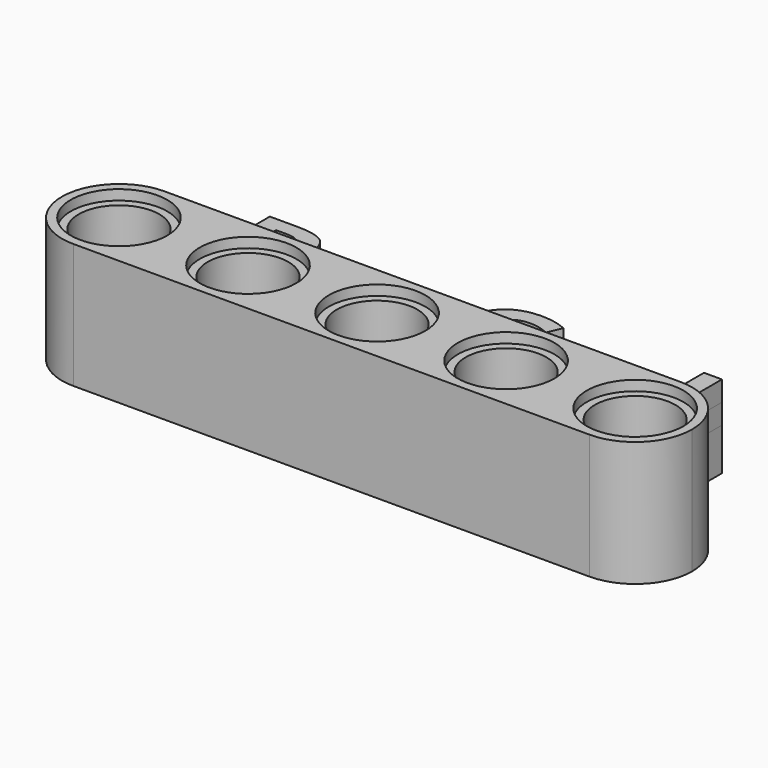
from build123d import *

# Parameters (mm, degrees)
F0_R         = 3.048
F0_R_2       = 2.54
F1_DEPTH     = 3.937
F2_R         = 3.0417071759
F3_DEPTH     = 0.635
F4_R         = 3.048
F5_DEPTH     = 0.635
F6_TEXT_SIZE = 7.5637000716
F7_DEPTH     = 3.937
F8_SIZE2     = 0.50799
F8_SIZE      = 0.50799
F9_SIZE2     = 0.50799
F9_SIZE      = 0.50799
F10_DEPTH    = 1.27


# Not quite as in the source:
# - a fillet or chamfer is up to 0.001 mm smaller than in the source, because OpenCascade refuses the exact size
# - Text() gives the source's letters only with a copy of the font that has no kerning and outlines rounded to 1/6400 em; it was checked with that copy


with BuildPart() as f1:
    # F0 (on Top) → F1 (new body, symmetric)
    with BuildSketch(Plane.XY):
        with BuildLine():
            ThreePointArc((-40.9946195992, 14.3710068385), (-42.0464330806, 16.9103092103), (-44.5857354524, 17.9621226917))
            ThreePointArc((-44.5857354524, 17.9621226917), (-48.1768513056, 14.3710068385), (-44.5857354524, 10.7798909853))
            ThreePointArc((-44.5857354524, 10.7798909853), (-42.0464330806, 11.8317044667), (-40.9946195992, 14.3710068385))
        make_face()
        with Locations((-44.5857354524, 14.3710068385)):
            Circle(F0_R, mode=Mode.SUBTRACT)
        with BuildLine():
            ThreePointArc((-49.1226195992, 14.3710068385), (-50.1744330806, 16.9103092103), (-52.7137354524, 17.9621226917))
            ThreePointArc((-52.7137354524, 17.9621226917), (-56.3048513056, 14.3710068385), (-52.7137354524, 10.7798909853))
            ThreePointArc((-52.7137354524, 10.7798909853), (-50.1744330806, 11.8317044667), (-49.1226195992, 14.3710068385))
        make_face()
        with Locations((-52.7137354524, 14.3710068385)):
            Circle(F0_R, mode=Mode.SUBTRACT)
        with BuildLine():
            ThreePointArc((-32.8666195992, 14.3710068385), (-33.9184330806, 16.9103092103), (-36.4577354524, 17.9621226917))
            ThreePointArc((-36.4577354524, 17.9621226917), (-40.0488513056, 14.3710068385), (-36.4577354524, 10.7798909853))
            ThreePointArc((-36.4577354524, 10.7798909853), (-33.9184330806, 11.8317044667), (-32.8666195992, 14.3710068385))
        make_face()
        with Locations((-36.4577354524, 14.3710068385)):
            Circle(F0_R, mode=Mode.SUBTRACT)
        with BuildLine():
            ThreePointArc((-24.7386195992, 14.3710068385), (-25.7904330806, 16.9103092103), (-28.3297354524, 17.9621226917))
            ThreePointArc((-28.3297354524, 17.9621226917), (-31.9208513056, 14.3710068385), (-28.3297354524, 10.7798909853))
            ThreePointArc((-28.3297354524, 10.7798909853), (-25.7904330806, 11.8317044667), (-24.7386195992, 14.3710068385))
        make_face()
        with Locations((-28.3297354524, 14.3710068385)):
            Circle(F0_R, mode=Mode.SUBTRACT)
        with BuildLine():
            ThreePointArc((-60.8417354524, 10.7798909853), (-58.3024330806, 11.8317044667), (-57.2506195992, 14.3710068385))
            ThreePointArc((-57.2506195992, 14.3710068385), (-58.3024330806, 16.9103092103), (-60.8417354524, 17.9621226917))
            ThreePointArc((-60.8417354524, 17.9621226917), (-64.4328513056, 14.3710068385), (-60.8417354524, 10.7798909853))
        make_face()
        with Locations((-60.8417354524, 14.3710068385)):
            Circle(F0_R, mode=Mode.SUBTRACT)
        with Locations((-44.5857354524, 14.3710068385)):
            Circle(F0_R)
        with Locations((-44.5857354524, 14.3710068385)):
            Circle(F0_R_2, mode=Mode.SUBTRACT)
        with Locations((-36.4577354524, 14.3710068385)):
            Circle(F0_R)
        with Locations((-36.4577354524, 14.3710068385)):
            Circle(F0_R_2, mode=Mode.SUBTRACT)
        with Locations((-52.7137354524, 14.3710068385)):
            Circle(F0_R)
        with Locations((-52.7137354524, 14.3710068385)):
            Circle(F0_R_2, mode=Mode.SUBTRACT)
        with Locations((-28.3297354524, 14.3710068385)):
            Circle(F0_R)
        with Locations((-28.3297354524, 14.3710068385)):
            Circle(F0_R_2, mode=Mode.SUBTRACT)
        with Locations((-60.8417354524, 14.3710068385)):
            Circle(F0_R)
        with Locations((-60.8417354524, 14.3710068385)):
            Circle(F0_R_2, mode=Mode.SUBTRACT)
        with BuildLine():
            ThreePointArc((-60.8417354524, 17.9621226917), (-58.3024330806, 16.9103092103), (-57.2506195992, 14.3710068385))
            ThreePointArc((-57.2506195992, 14.3710068385), (-58.3024330806, 11.8317044667), (-60.8417354524, 10.7798909853))
            Line((-60.8417354524, 10.7798909853), (-52.7137354524, 10.7798909853))
            ThreePointArc((-52.7137354524, 10.7798909853), (-56.3048513056, 14.3710068385), (-52.7137354524, 17.9621226917))
            Line((-52.7137354524, 17.9621226917), (-60.8417354524, 17.9621226917))
        make_face()
        with BuildLine():
            Line((-44.5857354524, 17.9621226917), (-52.7137354524, 17.9621226917))
            ThreePointArc((-52.7137354524, 17.9621226917), (-50.1744330806, 16.9103092103), (-49.1226195992, 14.3710068385))
            ThreePointArc((-49.1226195992, 14.3710068385), (-50.1744330806, 11.8317044667), (-52.7137354524, 10.7798909853))
            Line((-52.7137354524, 10.7798909853), (-44.5857354524, 10.7798909853))
            ThreePointArc((-44.5857354524, 10.7798909853), (-48.1768513056, 14.3710068385), (-44.5857354524, 17.9621226917))
        make_face()
        with BuildLine():
            Line((-28.3297354524, 17.9621226917), (-36.4577354524, 17.9621226917))
            ThreePointArc((-36.4577354524, 17.9621226917), (-33.9184330806, 16.9103092103), (-32.8666195992, 14.3710068385))
            ThreePointArc((-32.8666195992, 14.3710068385), (-33.9184330806, 11.8317044667), (-36.4577354524, 10.7798909853))
            Line((-36.4577354524, 10.7798909853), (-28.3297354524, 10.7798909853))
            ThreePointArc((-28.3297354524, 10.7798909853), (-31.9208513056, 14.3710068385), (-28.3297354524, 17.9621226917))
        make_face()
        with BuildLine():
            Line((-36.4577354524, 17.9621226917), (-44.5857354524, 17.9621226917))
            ThreePointArc((-44.5857354524, 17.9621226917), (-42.0464330806, 16.9103092103), (-40.9946195992, 14.3710068385))
            ThreePointArc((-40.9946195992, 14.3710068385), (-42.0464330806, 11.8317044667), (-44.5857354524, 10.7798909853))
            Line((-44.5857354524, 10.7798909853), (-36.4577354524, 10.7798909853))
            ThreePointArc((-36.4577354524, 10.7798909853), (-40.0488513056, 14.3710068385), (-36.4577354524, 17.9621226917))
        make_face()
    extrude(amount=F1_DEPTH, both=True)

    # F2 (on face) → F3 (cut)
    with BuildSketch(Plane.XY.offset(3.937)):
        with Locations((-28.3297354524, 14.3710068385)):
            Circle(F2_R)
        with Locations((-36.4577354524, 14.3710068385)):
            Circle(F2_R)
        with Locations((-44.5857354524, 14.3710068385)):
            Circle(F2_R)
        with Locations((-52.7137354524, 14.3710068385)):
            Circle(F2_R)
        with Locations((-60.8417354524, 14.3710068385)):
            Circle(F2_R)
    extrude(amount=-F3_DEPTH, mode=Mode.SUBTRACT)

    # F4 (on face) → F5 (cut)
    with BuildSketch(Plane(origin=(0, 0, -3.937), x_dir=(1, 0, 0), z_dir=(0, 0, -1))):
        with Locations((-60.8417354524, -14.3710068385)):
            Circle(F4_R)
        with Locations((-52.7137354524, -14.3710068385)):
            Circle(F4_R)
        with Locations((-44.5857354524, -14.3710068385)):
            Circle(F4_R)
        with Locations((-36.4577354524, -14.3710068385)):
            Circle(F4_R)
        with Locations((-28.3297354524, -14.3710068385)):
            Circle(F4_R)
    extrude(amount=-F5_DEPTH, mode=Mode.SUBTRACT)

    # F6 (on Top) → F7 (join)
    with BuildSketch(Plane.XY):
        with Locations((-59.0033847839, 17.6996979862)):
            Text('BenGod', F6_TEXT_SIZE, font='Open Sans', font_style=FontStyle.BOLD, text_align=(TextAlign.LEFT, TextAlign.BOTTOM))
    extrude(amount=-F7_DEPTH)

    # F8 (size 0.508 and 0.508 in the source; OpenCascade refuses exactly that, so slightly less here)
    f8_edges = [f1.edges().sort_by_distance(p)[0] for p in [
        (-38.997735, 14.371007, -3.302),
    ]]
    chamfer(f8_edges, length=F8_SIZE, length2=F8_SIZE2)

    # F9 (size 0.508 and 0.508 in the source; OpenCascade refuses exactly that, so slightly less here)
    f9_edges = [f1.edges().sort_by_distance(p)[0] for p in [
        (-47.125735, 14.371007, -3.302),
        (-55.253735, 14.371007, -3.302),
        (-63.381735, 14.371007, -3.302),
        (-30.869735, 14.371007, -3.302),
    ]]
    chamfer(f9_edges, length=F9_SIZE, length2=F9_SIZE2)

    # F6 (on Top) → F10 (join, symmetric)
    with BuildSketch(Plane.XY):
        with Locations((-59.0033847839, 17.6996979862)):
            Text('BenGod', F6_TEXT_SIZE, font='Open Sans', font_style=FontStyle.BOLD, text_align=(TextAlign.LEFT, TextAlign.BOTTOM))
    extrude(amount=F10_DEPTH, both=True)


solid = f1.part
